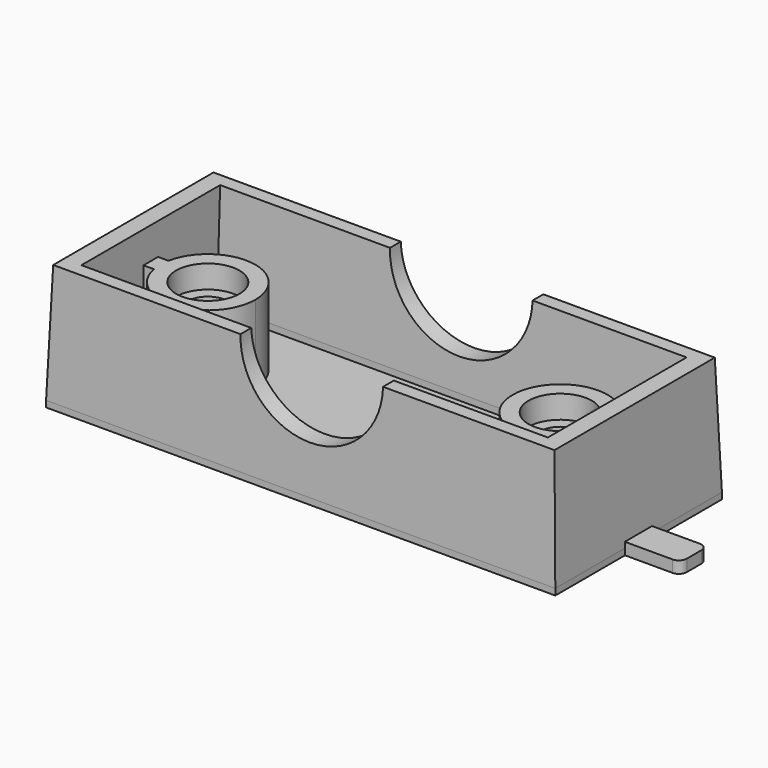
from build123d import *

# Parameters (mm, degrees)
F0_W         = 64.3
F0_H         = 26.3
F1_DEPTH     = 2
F2_W         = 64.3
F2_H         = 26.3
F2_W_2       = 58.9
F2_H_2       = 20.9
F3_DEPTH     = 13.8
F5_DEPTH     = 26.5
F7_DEPTH     = 9.8
F8_R         = 4
F9_DEPTH     = 2.9
F10_R        = 4
F11_DEPTH    = 2.9
F12_R        = 2.5
F13_DEPTH    = 9
F14_R        = 2.5
F15_DEPTH    = 9
F16_R        = 4.6
F17_DEPTH    = 7.2
F18_T1_DEPTH = 102.1483987537
F18_T3_DEPTH = 104.2983987537
F18_T5_DEPTH = 100.1483987537
F19_T1_DEPTH = 53.2490764557
F19_T3_DEPTH = 55.2490764557
F20_W        = 8.1560949282
F20_H        = 4.3
F21_DEPTH    = 1.5
F22_R        = 1


# Not quite as in the source:
# - a fillet or chamfer that OpenCascade refuses, or shapes differently, is made with other operations: its cross-section is extruded or revolved along the edge and cut away or added


with BuildPart() as f1:
    # F0 (on Top) → F1 (new body)
    with BuildSketch(Plane.XY):
        Rectangle(F0_W, F0_H)
    extrude(amount=F1_DEPTH)

    # F2 (on face) → F3 (join)
    with BuildSketch(Plane.XY.offset(2)):
        Rectangle(F2_W, F2_H)
        Rectangle(F2_W_2, F2_H_2, mode=Mode.SUBTRACT)
    extrude(amount=F3_DEPTH)

    # F4 (on face) → F5 (cut)
    with BuildSketch(Plane.XZ.offset(13.15)):
        with BuildLine():
            ThreePointArc((-8, 15.8), (1, 6.8), (10, 15.8))
            Line((10, 15.8), (-8, 15.8))
        make_face()
    extrude(amount=-F5_DEPTH, mode=Mode.SUBTRACT)

    # F6 (on face) → F7 (join)
    with BuildSketch(Plane.XY.offset(2)):
        with BuildLine():
            ThreePointArc((-28.1387604808, -1.15), (-21.6723162131, -5.9721253706), (-16.25, 0))
            ThreePointArc((-16.25, 0), (-21.6723162131, 5.9721253706), (-28.1387604808, 1.15))
            Line((-28.1387604808, 1.15), (-28.1387604808, -1.15))
        make_face()
        with BuildLine():
            Line((-28.1387604808, -1.15), (-28.1387604808, 1.15))
            ThreePointArc((-28.1387604808, 1.15), (-28.25, 0), (-28.1387604808, -1.15))
        make_face()
        with BuildLine():
            ThreePointArc((-28.1387604808, -1.15), (-28.25, 0), (-28.1387604808, 1.15))
            Line((-28.1387604808, 1.15), (-30.8787655085, 1.15))
            Line((-30.8787655085, 1.15), (-30.8787655085, -1.15))
            Line((-30.8787655085, -1.15), (-29.45, -1.15))
            Line((-29.45, -1.15), (-28.1387604808, -1.15))
        make_face()
        with BuildLine():
            ThreePointArc((28.1387604808, -1.15), (28.2221253706, -0.5776837869), (28.25, 0))
            ThreePointArc((28.25, 0), (28.2221253706, 0.5776837869), (28.1387604808, 1.15))
            Line((28.1387604808, 1.15), (28.1387604808, -1.15))
        make_face()
        with BuildLine():
            ThreePointArc((28.1387604808, 1.15), (28.2221253706, 0.5776837869), (28.25, 0))
            ThreePointArc((28.25, 0), (28.2221253706, -0.5776837869), (28.1387604808, -1.15))
            Line((28.1387604808, -1.15), (29.9528725445, -1.15))
            Line((29.9528725445, -1.15), (29.9528725445, 1.15))
            Line((29.9528725445, 1.15), (28.1387604808, 1.15))
        make_face()
        with BuildLine():
            Line((28.1387604808, -1.15), (28.1387604808, 1.15))
            ThreePointArc((28.1387604808, 1.15), (16.25, 0), (28.1387604808, -1.15))
        make_face()
    extrude(amount=F7_DEPTH)

    # F8 (on face) → F9 (cut)
    with BuildSketch(Plane.XY.offset(11.8)):
        with Locations((-22.25, 0)):
            Circle(F8_R)
    extrude(amount=-F9_DEPTH, mode=Mode.SUBTRACT)

    # F10 (on face) → F11 (cut)
    with BuildSketch(Plane.XY.offset(11.8)):
        with Locations((22.25, 0)):
            Circle(F10_R)
    extrude(amount=-F11_DEPTH, mode=Mode.SUBTRACT)

    # F12 (on face) → F13 (cut)
    with BuildSketch(Plane.XY.offset(8.9)):
        with Locations((-22.25, 0)):
            Circle(F12_R)
    extrude(amount=-F13_DEPTH, mode=Mode.SUBTRACT)

    # F14 (on face) → F15 (cut)
    with BuildSketch(Plane.XY.offset(8.9)):
        with Locations((22.25, 0)):
            Circle(F14_R)
    extrude(amount=-F15_DEPTH, mode=Mode.SUBTRACT)

    # F16 (on face) → F17 (cut)
    with BuildSketch(Plane(origin=(0, 0, 0), x_dir=(1, 0, 0), z_dir=(0, 0, -1))):
        with Locations((-22.25, 0)):
            Circle(F16_R)
        with Locations((22.25, 0)):
            Circle(F16_R)
    extrude(amount=-F17_DEPTH, mode=Mode.SUBTRACT)

    # F18: chamfer of 15 x 0.5 on 6 edges, made by hand

    # F18_s2 → F18_t1 (cut)
    with BuildSketch(Plane.YZ.offset(-71.1491993768)):
        Polygon((13.15, 0.8), (12.65, 15.8), (13.15, 15.8), align=None)
        Polygon((-12.65, 15.8), (-13.15, 0.8), (-13.15, 15.8), align=None)
    extrude(amount=F18_T1_DEPTH, mode=Mode.SUBTRACT)

    # F18_s4 → F18_t3 (cut)
    with BuildSketch(Plane.XZ.offset(-52.1491993768)):
        Polygon((32.15, 0.8), (31.65, 15.8), (32.15, 15.8), align=None)
        Polygon((-32.15, 0.8), (-31.65, 15.8), (-32.15, 15.8), align=None)
    extrude(amount=F18_T3_DEPTH, mode=Mode.SUBTRACT)

    # F18_s6 → F18_t5 (cut)
    with BuildSketch(Plane.YZ.offset(-28.9991993768)):
        Polygon((13.15, 0.8), (12.65, 15.8), (13.15, 15.8), align=None)
        Polygon((-12.65, 15.8), (-13.15, 0.8), (-13.15, 15.8), align=None)
    extrude(amount=F18_T5_DEPTH, mode=Mode.SUBTRACT)

    # F19: chamfer of 13 x 0.5 on 4 edges, made by hand

    # F19_s2 → F19_t1 (cut)
    with BuildSketch(Plane.YZ.offset(-23.7990764557)):
        Polygon((-10.95, 15.8), (-10.45, 2.8), (-10.45, 15.8), align=None)
        Polygon((10.45, 2.8), (10.95, 15.8), (10.45, 15.8), align=None)
    extrude(amount=F19_T1_DEPTH, mode=Mode.SUBTRACT)

    # F19_s4 → F19_t3 (cut)
    with BuildSketch(Plane.YZ.offset(-29.45)):
        Polygon((10.45, 2.8), (10.95, 15.8), (10.45, 15.8), align=None)
        Polygon((-10.95, 15.8), (-10.45, 2.8), (-10.45, 15.8), align=None)
    extrude(amount=F19_T3_DEPTH, mode=Mode.SUBTRACT)

    # F20 (on Top) → F21 (join)
    with BuildSketch(Plane.XY):
        with Locations((35.0719525359, 0)):
            Rectangle(F20_W, F20_H)
    extrude(amount=F21_DEPTH)

    # F22
    f22_edges = [f1.edges().sort_by_distance(p)[0] for p in [
        (39.15, 2.15, 0.75),
        (39.15, -2.15, 0.75),
    ]]
    fillet(f22_edges, radius=F22_R)


solid = f1.part
